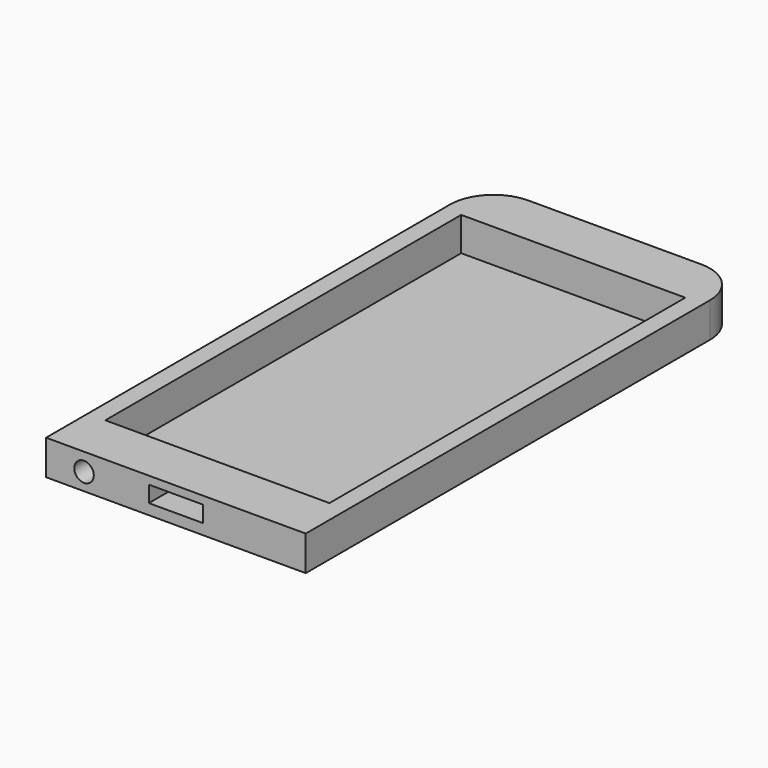
from build123d import *

# Parameters (mm, degrees)
F0_W     = 50.6464093924
F0_H     = 100.5250141025
F1_DEPTH = 0.254
F0_W_2   = 58.674
F0_H_2   = 123.952
F2_DEPTH = 7.874
F3_R     = 9.8113639175
F4_R     = 9.8044
F6_W     = 12.2285038233
F6_H     = 3.6733425222
F7_DEPTH = 17.272
F8_R     = 2.2102361545
F9_DEPTH = 12.192


# Not quite as in the source:
# - the program builds the solid bodies; features that only make, move or delete a surface that nothing else refers to are left out


with BuildPart() as f1:
    # F0 (on Top) → F1 (new body)
    with BuildSketch(Plane.XY):
        with Locations((55.8215677738, 54.941402014)):
            Rectangle(F0_W, F0_H)
    extrude(amount=F1_DEPTH)

    # F0 (on Top) → F2 (join)
    with BuildSketch(Plane.XY):
        with Locations((55.8215677738, 54.941402014)):
            Rectangle(F0_W_2, F0_H_2)
        with Locations((55.8215677738, 54.941402014)):
            Rectangle(F0_W, F0_H, mode=Mode.SUBTRACT)
    extrude(amount=F2_DEPTH)

    # F3
    f3_edges = [f1.edges().sort_by_distance(p)[0] for p in [
        (26.484568, 116.917402, 3.937),
    ]]
    fillet(f3_edges, radius=F3_R)

    # F4
    f4_edges = [f1.edges().sort_by_distance(p)[0] for p in [
        (85.158568, 116.917402, 3.937),
    ]]
    fillet(f4_edges, radius=F4_R)

    # F6 (on face) → F7 (cut)
    with BuildSketch(Plane.XZ.offset(7.034597986)):
        with Locations((55.8215677738, 4.2473026551)):
            Rectangle(F6_W, F6_H)
    extrude(amount=-F7_DEPTH, mode=Mode.SUBTRACT)

    # F8 (on face) → F9 (cut)
    with BuildSketch(Plane.XZ.offset(7.034597986)):
        with Locations((35.0567772985, 3.8737377618)):
            Circle(F8_R)
    extrude(amount=-F9_DEPTH, mode=Mode.SUBTRACT)


solid = f1.part
